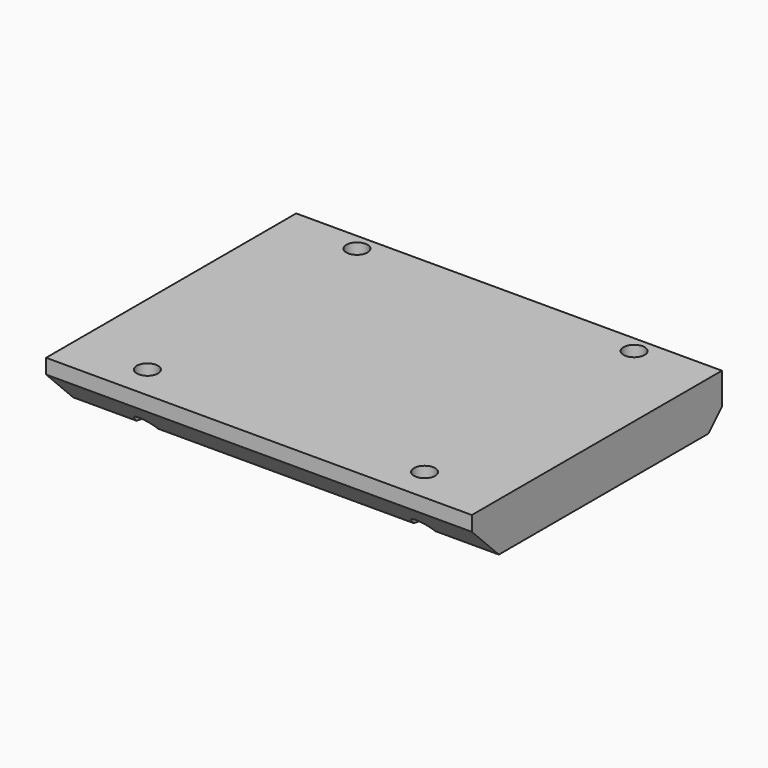
from build123d import *

# Parameters (mm, degrees)
F0_W        = 159.9819
F0_H        = 117.475
F1_DEPTH    = 18.25625
F3_D        = 7.9375
F5_D        = 7.9375
F6_T1_DEPTH = 225.3026478943
F7_T1_DEPTH = 192.6422739472


# Not quite as in the source:
# - a fillet or chamfer that OpenCascade refuses, or shapes differently, is made with other operations: its cross-section is extruded or revolved along the edge and cut away or added


with BuildPart() as f1:
    # F0 (on Top) → F1 (new body)
    with BuildSketch(Plane.XY):
        with Locations((79.99095, 58.7375)):
            Rectangle(F0_W, F0_H)
    extrude(amount=F1_DEPTH)

    # F3 (through all)
    with Locations(Plane.XY.offset(18.25625)):
        with Locations((27.90825, 12.7), (132.07365, 12.7)):
            Hole(F3_D / 2)

    # F5 (through all)
    with Locations(Plane.XY.offset(18.25625)):
        with Locations((27.90825, 111.125), (132.07365, 111.125)):
            Hole(F5_D / 2)

    # F6: chamfer of 12.7 on 1 edges, made by hand

    # F6_s2 → F6_t1 (cut)
    with BuildSketch(Plane.YZ.offset(-32.6603739472)):
        Polygon((0, 12.7), (12.7, 0), (0, 0), align=None)
    extrude(amount=F6_T1_DEPTH, mode=Mode.SUBTRACT)

    # F7: chamfer of 6.35 on 1 edges, made by hand

    # F7_s2 → F7_t1 (cut)
    with BuildSketch(Plane.YZ.offset(-16.3301869736)):
        Polygon((111.125, 0), (117.475, 6.35), (117.475, 0), align=None)
    extrude(amount=F7_T1_DEPTH, mode=Mode.SUBTRACT)


solid = f1.part
